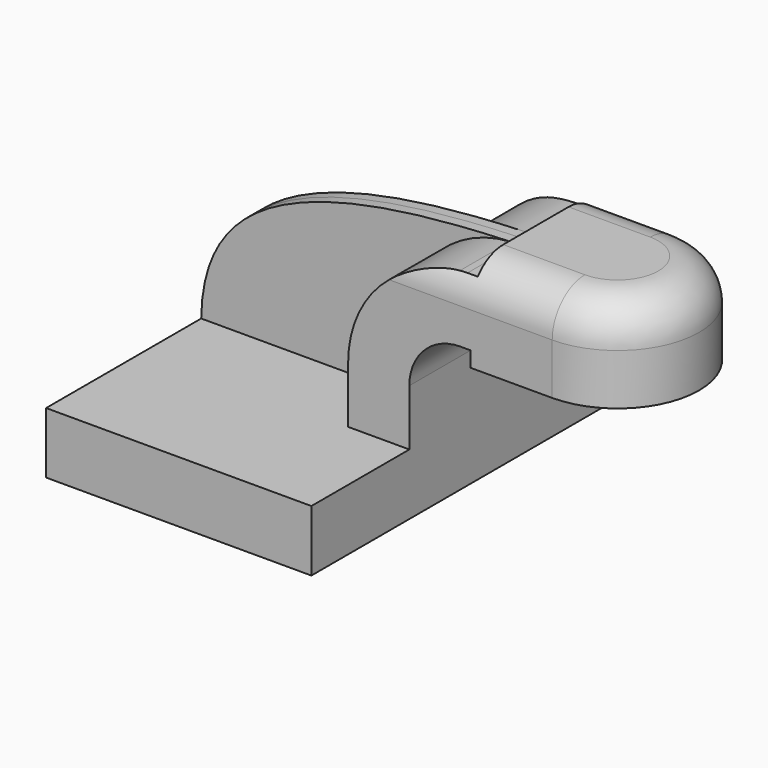
from build123d import *

# Parameters (mm, degrees)
F1_DEPTH = 63.5
F0_W     = 25.4
F0_H     = 19.05
F0_H_2   = 4.7498
F0_H_3   = 4.7752
F2_DEPTH = 25.4
F4_DEPTH = 3.175
F5_R     = 12.7


with BuildPart() as f1:
    # F0 (on Front) → F1 (new body, symmetric)
    with BuildSketch(Plane.XZ):
        Polygon((-41.275, 9.525), (-41.275, -9.525), (41.275, -9.525), (41.275, 9.525), (22.225, 9.525), align=None)
    extrude(amount=F1_DEPTH, both=True)

    # F0 (on Front) → F2 (join, symmetric)
    with BuildSketch(Plane.XZ):
        with BuildLine():
            Line((22.225, 9.525), (41.275, 9.525))
            Line((41.275, 9.525), (41.275, 27.0002))
            ThreePointArc((41.275, 27.0002), (45.9246798487, 38.2255201513), (57.15, 42.8752))
            Line((57.15, 42.8752), (60.325, 42.8752))
            Line((60.325, 42.8752), (60.325, 61.9252))
            Line((60.325, 61.9252), (57.15, 61.9252))
            add(Edge.make_bspline(
                [(54.8690383613, 61.8506352771), (55.6242381587, 61.8771737888), (56.3845511944, 61.9020277216), (57.15, 61.9252)],
                knots=[110.3049530316, 110.3049530316, 110.3049530316, 110.3049530316, 111.5045361635, 111.5045361635, 111.5045361635, 111.5045361635], degree=3))
            ThreePointArc((54.8690383613, 61.8506352771), (31.6606079885, 50.8758470045), (22.225, 27.0002))
            Line((22.225, 27.0002), (22.225, 9.525))
        make_face()
        with Locations((73.025, 52.4002)):
            Rectangle(F0_W, F0_H)
        with Locations((73.025, 64.3001)):
            Rectangle(F0_W, F0_H_2)
        with Locations((73.025, 40.4876)):
            Rectangle(F0_W, F0_H_3)
    extrude(amount=F2_DEPTH, both=True)

    # F0 (on Front) → F3 (revolve)
    with BuildSketch(Plane.XZ):
        Polygon((85.725, 66.675), (85.725, 61.9252), (85.725, 42.8752), (85.725, 38.1), (111.125, 38.1), (111.125, 66.675), align=None)
    revolve(axis=Axis((85.725, 0, 52.3875), (0, 0, 1)))

    # F0 (on Front) → F4 (join, symmetric)
    with BuildSketch(Plane.XZ):
        with BuildLine():
            add(Edge.make_bspline(
                [(-41.275, 9.525), (-40.782344334, 42.7264267902), (-14.5736504872, 59.4103464678), (54.8690383613, 61.8506352771)],
                knots=[0, 0, 0, 0, 110.3049530316, 110.3049530316, 110.3049530316, 110.3049530316], degree=3))
            Line((-41.275, 9.525), (22.225, 9.525))
            Line((22.225, 9.525), (22.225, 27.0002))
            ThreePointArc((22.225, 27.0002), (31.6606079885, 50.8758470045), (54.8690383613, 61.8506352771))
        make_face()
    extrude(amount=F4_DEPTH, both=True)

    # F5
    f5_edges = [f1.edges().sort_by_distance(p)[0] for p in [
        (85.725, 25.4, 52.3875),
        (73.025, -25.4, 66.675),
        (73.025, 25.4, 66.675),
        (111.125, 0, 66.675),
    ]]
    fillet(f5_edges, radius=F5_R)


solid = f1.part
